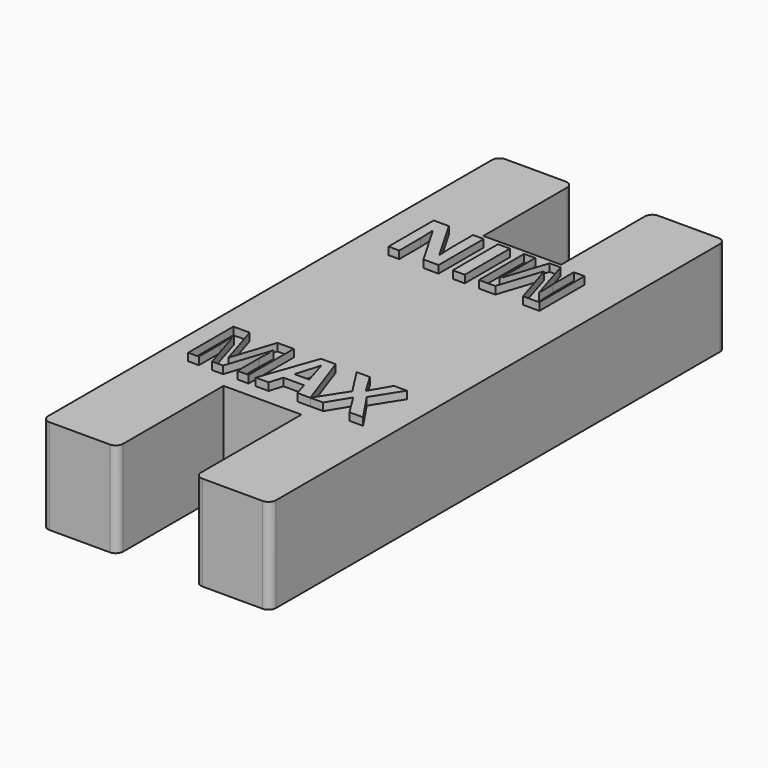
from build123d import *

# Parameters (mm, degrees)
F1_DEPTH     = 12.7
F2_TEXT_SIZE = 10.5833333333
F3_DEPTH     = 1.016
F4_R         = 0.9906


# Not quite as in the source:
# - Text() gives the source's letters only with a copy of the font that has no kerning and outlines rounded to 1/6400 em; it was checked with that copy


with BuildPart() as f1:
    # F0 (on Top) → F1 (new body)
    with BuildSketch(Plane.XY):
        Polygon((-5.207, 38.1), (-15.24, 38.1), (-15.24, -38.1), (-5.207, -38.1), (-5.207, -20.32), (5.207, -20.32), (5.207, -38.1), (15.24, -38.1), (15.24, 38.1), (5.207, 38.1), (5.207, 23.114), (-5.207, 23.114), align=None)
    extrude(amount=F1_DEPTH)

    # F4
    f4_edges = [f1.edges().sort_by_distance(p)[0] for p in [
        (5.207, 38.1, 6.35),
        (-5.207, 38.1, 6.35),
        (-15.24, 38.1, 6.35),
        (15.24, 38.1, 6.35),
        (-15.24, -38.1, 6.35),
        (-5.207, -38.1, 6.35),
        (5.207, -38.1, 6.35),
        (15.24, -38.1, 6.35),
    ]]
    fillet(f4_edges, radius=F4_R)


with BuildPart() as f3:
    # F2 (on face) → F3 (new body)
    with BuildSketch(Plane.XY.offset(12.7)):
        with Locations((-12.5131380208, -18.288)):
            Text('MAX', F2_TEXT_SIZE, font='Open Sans', font_style=FontStyle.BOLD, text_align=(TextAlign.LEFT, TextAlign.BOTTOM))
        with Locations(Location((10.9107552083, 21.082), (0, 0, -180))):
            Text('MIN', F2_TEXT_SIZE, font='Open Sans', font_style=FontStyle.BOLD, text_align=(TextAlign.LEFT, TextAlign.BOTTOM))
    extrude(amount=F3_DEPTH)


solid = Compound([f1.part, f3.part])
